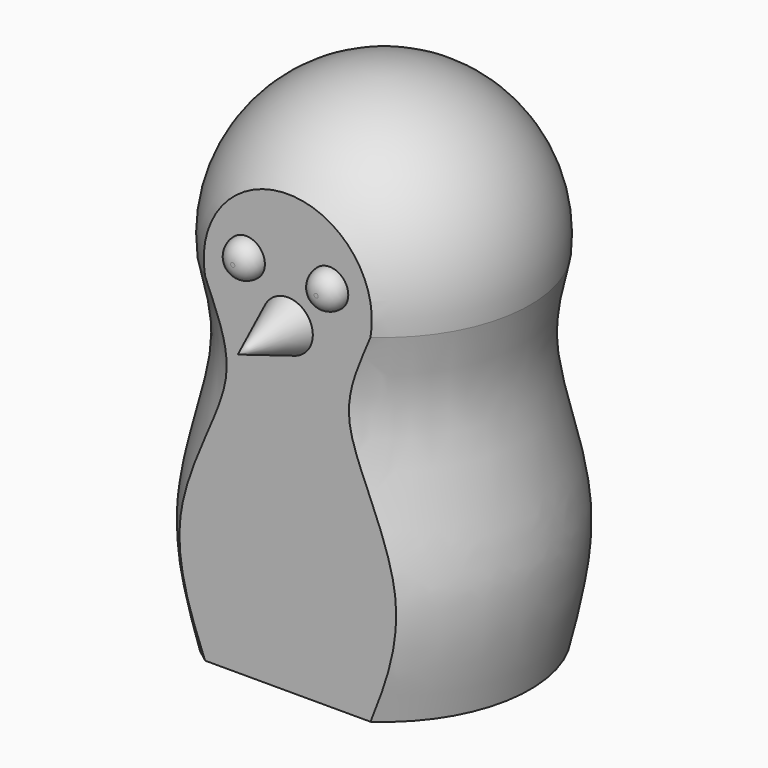
from build123d import *

# Parameters (mm, degrees)
F3_DEPTH  = 177.8
F4_R      = 7.62
F5_DEPTH  = 19.05
F6_SIZE2  = 18.860161823
F6_SIZE   = 7.62
F4_R_2    = 5.715
F7_DEPTH  = 5.08
F8_R      = 5.07999
F9_R      = 6.35
F10_DEPTH = 50.8
F11_SCALE = 1.1422


# Not quite as in the source:
# - a fillet or chamfer is up to 0.001 mm smaller than in the source, because OpenCascade refuses the exact size


with BuildPart() as f1:
    # F0 (on Front) → F1 (revolve)
    with BuildSketch(Plane.XZ):
        with BuildLine():
            Line((-38.2711647941, 0), (0, 0))
            Line((0, 0), (0, 146.0500033258))
            Line((0, 146.0500033258), (0, 152.4))
            ThreePointArc((0, 152.4), (-33.2006597867, 137.6319951518), (-44.4655865431, 103.0852268133))
            add(Edge.make_bspline(
                [(-44.4655865431, 0), (-47.1114422222, 11.762074058), (-53.3469479224, 35.8297600734), (-37.8272166921, 76.0482431769), (-42.543614325, 94.8604386904), (-44.4655865431, 103.0852268133)],
                knots=[0, 0, 0, 0, 0.3424224234, 0.7066775859, 1, 1, 1, 1], degree=3))
            Line((-44.4655865431, 0), (-38.2711647941, 0))
        make_face()
    revolve(axis=Axis((0, 0, 76.2), (0, 0, 1)))

    # F2 (on Top) → F3 (cut)
    with BuildSketch(Plane.XY):
        Polygon((25.6092443837, -36.641700535), (-25.1907556163, -36.641700535), (-46.7807556163, -36.641700535), (-46.7807556163, -67.121700535), (42.1192443837, -67.121700535), (42.1192443837, -36.641700535), align=None)
    extrude(amount=F3_DEPTH, mode=Mode.SUBTRACT)

    # F4 (on face) → F5 (join)
    with BuildSketch(Plane.XZ.offset(36.641700535)):
        with Locations((0, 97.9992443837)):
            Circle(F4_R)
    extrude(amount=F5_DEPTH)

    # F6
    f6_edges = [f1.edges().sort_by_distance(p)[0] for p in [
        (-7.62, -55.691701, 97.999244),
    ]]
    f6_side = f1.faces().sort_by_distance((0, -55.691701, 97.999244))[0]
    chamfer(f6_edges, length=F6_SIZE, length2=F6_SIZE2, reference=f6_side)

    # F4 (on face) → F7 (join)
    with BuildSketch(Plane.XZ.offset(36.641700535)):
        with Locations((-12.7, 112.2232443837)):
            Circle(F4_R_2)
        with Locations((12.7, 112.2232443837)):
            Circle(F4_R_2)
    extrude(amount=F7_DEPTH)

    # F8 (radius 5.08 in the source; OpenCascade refuses exactly that, so slightly less here)
    f8_edges = [f1.edges().sort_by_distance(p)[0] for p in [
        (-18.415, -41.721701, 112.223244),
        (6.985, -41.721701, 112.223244),
    ]]
    fillet(f8_edges, radius=F8_R)

    # F9 (on face) → F10 (cut)
    with BuildSketch(Plane(origin=(0, 0, 0), x_dir=(1, 0, 0), z_dir=(0, 0, -1))):
        Circle(F9_R)
    extrude(amount=-F10_DEPTH, mode=Mode.SUBTRACT)


with BuildPart() as f1_1:
    # F11: moved
    add(f1.part.scale(F11_SCALE))


solid = f1_1.part
